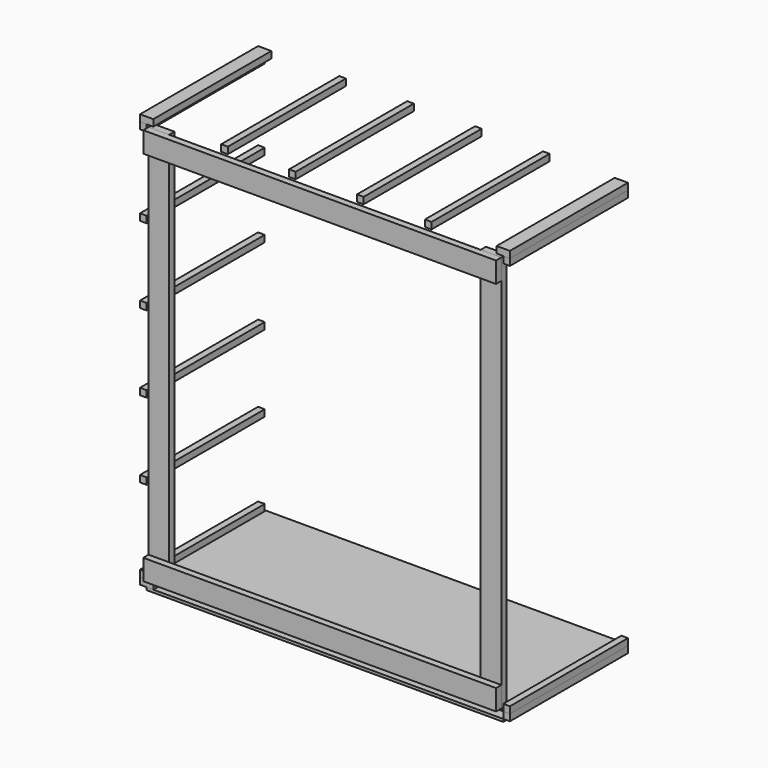
from build123d import *

# Parameters (mm, degrees)
F0_W     = 140
F0_H     = 140
F0_H_2   = 2410
F1_DEPTH = 45
F0_W_2   = 2110
F2_DEPTH = 45
F3_DEPTH = 1000
F0_W_3   = 45
F0_H_3   = 45
F4_DEPTH = 1000
F5_DEPTH = 1000
F6_DEPTH = 1000
F7_DEPTH = 1000
F8_DEPTH = 1000


with BuildPart() as f1:
    # F0 (on Front) → F1 (new body)
    with BuildSketch(Plane.XZ):
        with Locations((75, 75)):
            Rectangle(F0_W, F0_H)
        with Locations((75, 1350)):
            Rectangle(F0_W, F0_H_2)
        with Locations((75, 2625)):
            Rectangle(F0_W, F0_H)
    extrude(amount=-F1_DEPTH)


with BuildPart() as f1b:
    # F0 (on Front) → F1, piece 2 (new body)
    with BuildSketch(Plane.XZ):
        with Locations((2325, 75)):
            Rectangle(F0_W, F0_H)
        with Locations((2325, 1350)):
            Rectangle(F0_W, F0_H_2)
        with Locations((2325, 2625)):
            Rectangle(F0_W, F0_H)
    extrude(amount=-F1_DEPTH)


with BuildPart() as f2:
    # F0 (on Front) → F2 (new body)
    with BuildSketch(Plane.XZ):
        with Locations((75, 75)):
            Rectangle(F0_W, F0_H)
        with Locations((1200, 75)):
            Rectangle(F0_W_2, F0_H)
        with Locations((2325, 75)):
            Rectangle(F0_W, F0_H)
    extrude(amount=F2_DEPTH)


with BuildPart() as f2b:
    # F0 (on Front) → F2, piece 2 (new body)
    with BuildSketch(Plane.XZ):
        with Locations((75, 2625)):
            Rectangle(F0_W, F0_H)
        with Locations((1200, 2625)):
            Rectangle(F0_W_2, F0_H)
        with Locations((2325, 2625)):
            Rectangle(F0_W, F0_H)
    extrude(amount=F2_DEPTH)


with BuildPart() as f3:
    # F0 (on Front) → F3 (new body)
    with BuildSketch(Plane.XZ):
        Polygon((37, -8), (0, -8), (-8, -8), (-53, -8), (-53, -53), (-8, -53), (37, -53), align=None)
    extrude(amount=-F3_DEPTH)


with BuildPart() as f3b:
    # F0 (on Front) → F3, piece 2 (new body)
    with BuildSketch(Plane.XZ):
        Polygon((-8, 2708), (0, 2708), (37, 2708), (37, 2753), (-8, 2753), align=None)
        with Locations((-30.5, 2730.5)):
            Rectangle(F0_W_3, F0_H_3)
    extrude(amount=-F3_DEPTH)


with BuildPart() as f3c:
    # F0 (on Front) → F3, piece 3 (new body)
    with BuildSketch(Plane.XZ):
        with Locations((2430.5, -30.5)):
            Rectangle(F0_W_3, F0_H_3)
    extrude(amount=-F3_DEPTH)


with BuildPart() as f3d:
    # F0 (on Front) → F3, piece 4 (new body)
    with BuildSketch(Plane.XZ):
        Polygon((2363, 2708), (2400, 2708), (2408, 2708), (2408, 2753), (2363, 2753), align=None)
        with Locations((2430.5, 2730.5)):
            Rectangle(F0_W_3, F0_H_3)
    extrude(amount=-F3_DEPTH)


with BuildPart() as f4:
    # F0 (on Front) → F4 (new body)
    with BuildSketch(Plane.XZ):
        with Locations((-30.5, 2685.5)):
            Rectangle(F0_W_3, F0_H_3)
    extrude(amount=-F4_DEPTH)


with BuildPart() as f4b:
    # F0 (on Front) → F4, piece 2 (new body)
    with BuildSketch(Plane.XZ):
        with Locations((2430.5, 2685.5)):
            Rectangle(F0_W_3, F0_H_3)
    extrude(amount=-F4_DEPTH)


with BuildPart() as f4c:
    # F0 (on Front) → F4, piece 3 (new body)
    with BuildSketch(Plane.XZ):
        with Locations((2430.5, 14.5)):
            Rectangle(F0_W_3, F0_H_3)
    extrude(amount=-F4_DEPTH)


with BuildPart() as f4d:
    # F0 (on Front) → F4, piece 4 (new body)
    with BuildSketch(Plane.XZ):
        with Locations((-30.5, 14.5)):
            Rectangle(F0_W_3, F0_H_3)
    extrude(amount=-F4_DEPTH)


with BuildPart() as f5:
    # F0 (on Front) → F5 (new body)
    with BuildSketch(Plane.XZ):
        Polygon((2354.4380664825, -53), (37, -53), (-8, -53), (-8, -71), (2408, -71), (2408, -53), align=None)
    extrude(amount=-F5_DEPTH)


with BuildPart() as f6:
    # F0 (on Front) → F6 (new body)
    with BuildSketch(Plane.XZ):
        Polygon((145, 0), (0, 0), (0, -8), (37, -8), (2354.4380664825, -8), (2400, -8), (2400, 0), (2255, 0), align=None)
    extrude(amount=-F6_DEPTH)


with BuildPart() as f7:
    # F0 (on Front) → F7 (new body)
    with BuildSketch(Plane.XZ):
        with Locations((519.5, 2730.5)):
            Rectangle(F0_W_3, F0_H_3)
    extrude(amount=-F7_DEPTH)


with BuildPart() as f7b:
    # F0 (on Front) → F7, piece 2 (new body)
    with BuildSketch(Plane.XZ):
        with Locations((979.5, 2730.5)):
            Rectangle(F0_W_3, F0_H_3)
    extrude(amount=-F7_DEPTH)


with BuildPart() as f7c:
    # F0 (on Front) → F7, piece 3 (new body)
    with BuildSketch(Plane.XZ):
        with Locations((1439.5, 2730.5)):
            Rectangle(F0_W_3, F0_H_3)
    extrude(amount=-F7_DEPTH)


with BuildPart() as f7d:
    # F0 (on Front) → F7, piece 4 (new body)
    with BuildSketch(Plane.XZ):
        with Locations((1899.5, 2730.5)):
            Rectangle(F0_W_3, F0_H_3)
    extrude(amount=-F7_DEPTH)


with BuildPart() as f8:
    # F0 (on Front) → F8 (new body)
    with BuildSketch(Plane.XZ):
        with Locations((-30.5, 579.5)):
            Rectangle(F0_W_3, F0_H_3)
    extrude(amount=-F8_DEPTH)


with BuildPart() as f8b:
    # F0 (on Front) → F8, piece 2 (new body)
    with BuildSketch(Plane.XZ):
        with Locations((-30.5, 1099.5)):
            Rectangle(F0_W_3, F0_H_3)
    extrude(amount=-F8_DEPTH)


with BuildPart() as f8c:
    # F0 (on Front) → F8, piece 3 (new body)
    with BuildSketch(Plane.XZ):
        with Locations((-30.5, 1619.5)):
            Rectangle(F0_W_3, F0_H_3)
    extrude(amount=-F8_DEPTH)


with BuildPart() as f8d:
    # F0 (on Front) → F8, piece 4 (new body)
    with BuildSketch(Plane.XZ):
        with Locations((-30.5, 2139.5)):
            Rectangle(F0_W_3, F0_H_3)
    extrude(amount=-F8_DEPTH)


solid = Compound([f1.part, f1b.part, f2.part, f2b.part, f3.part, f3b.part, f3c.part, f3d.part, f4.part, f4b.part, f4c.part, f4d.part, f5.part, f6.part, f7.part, f7b.part, f7c.part, f7d.part, f8.part, f8b.part, f8c.part, f8d.part])
